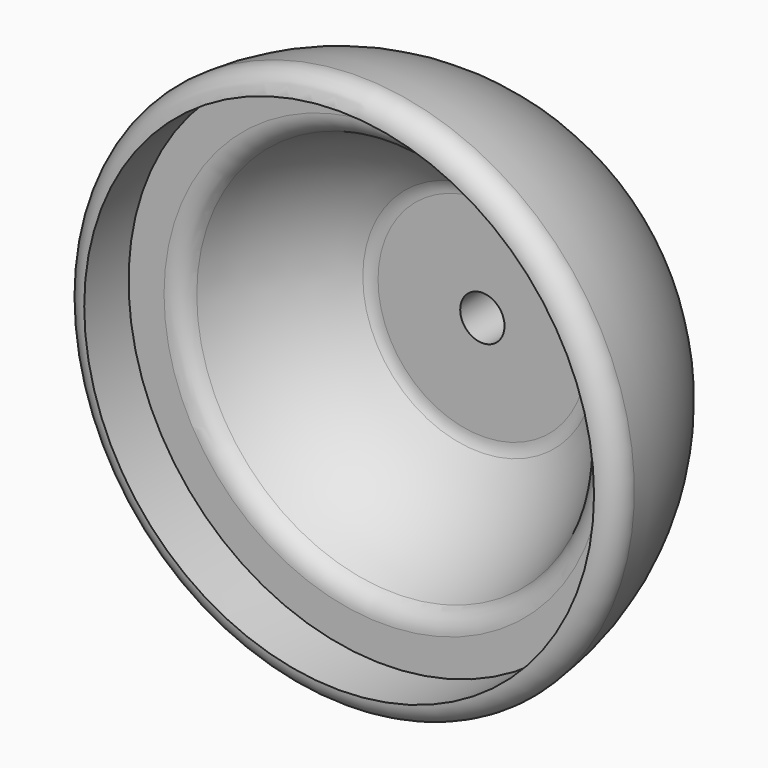
from build123d import *

# Parameters (mm, degrees)
F2_R      = 9
F2_R_2    = 6.5
F3_DEPTH  = 1
F4_R      = 5
F5_DEPTH  = 1
F6_R      = 23
F7_DEPTH  = 5
F8_R      = 2.5
F9_DEPTH  = 2
F10_R     = 2
F11_DEPTH = 25


# Not quite as in the source:
# - a fillet or chamfer that OpenCascade refuses, or shapes differently, is made with other operations: its cross-section is extruded or revolved along the edge and cut away or added


with BuildPart() as f1:
    # F0 (on Top) → F1 (revolve)
    with BuildSketch(Plane.XY):
        with BuildLine():
            ThreePointArc((-30.0702019767, 18.8458363465), (-40.98670264, 9.6260218093), (-45.0702019767, -4.0670421283))
            Line((-45.0702019767, -4.0670421283), (-39.0702019767, -4.0670421283))
            ThreePointArc((-39.0702019767, -4.0670421283), (-36.6683946494, 5.1795788761), (-30.0702019767, 12.0884522931))
            ThreePointArc((-30.0702019767, 12.0884522931), (-25.2685481557, 14.2080008813), (-20.0702019767, 14.9329578717))
            Line((-20.0702019767, 14.9329578717), (-20.0702019767, 18.8458363465))
            Line((-20.0702019767, 18.8458363465), (-30.0702019767, 18.8458363465))
        make_face()
        with BuildLine():
            ThreePointArc((-20.0702019767, 14.9329578717), (-25.2685481557, 14.2080008813), (-30.0702019767, 12.0884522931))
            Line((-30.0702019767, 12.0884522931), (-20.0702019767, 12.0884522931))
            Line((-20.0702019767, 12.0884522931), (-20.0702019767, 14.9329578717))
        make_face()
    revolve(axis=Axis((-20.0702019767, 9.4528388078, 0), (0, 1, 0)))

    # F2 (on face) → F3 (cut)
    with BuildSketch(Plane(origin=(0, 18.8458363465, 0), x_dir=(-1, 0, 0), z_dir=(0, 1, 0))):
        with Locations((20.0702019767, 0)):
            Circle(F2_R)
        with Locations((20.0702019767, 0)):
            Circle(F2_R_2, mode=Mode.SUBTRACT)
    extrude(amount=-F3_DEPTH, mode=Mode.SUBTRACT)

    # F4 (on face) → F5 (cut)
    with BuildSketch(Plane(origin=(0, 18.8458363465, 0), x_dir=(-1, 0, 0), z_dir=(0, 1, 0))):
        with Locations((20.0702019767, 0)):
            Circle(F4_R)
    extrude(amount=-F5_DEPTH, mode=Mode.SUBTRACT)

    # F6 (on face) → F7 (cut)
    with BuildSketch(Plane.XZ.offset(4.0670421283)):
        with Locations((-20.0702019767, 0)):
            Circle(F6_R)
    extrude(amount=-F7_DEPTH, mode=Mode.SUBTRACT)

    # F8 (on face) → F9 (join)
    with BuildSketch(Plane(origin=(0, 17.8458363465, 0), x_dir=(-1, 0, 0), z_dir=(0, 1, 0))):
        with Locations((20.0702019767, 0)):
            Circle(F8_R)
    extrude(amount=F9_DEPTH)

    # F10 (on face) → F11 (cut)
    with BuildSketch(Plane(origin=(0, 19.8458363465, 0), x_dir=(-1, 0, 0), z_dir=(0, 1, 0))):
        with Locations((20.0702019767, 0)):
            Circle(F10_R)
    extrude(amount=-F11_DEPTH, mode=Mode.SUBTRACT)

    # F12: fillet of radius 2 on 3 edges, made by hand

    # F12_s1 → F12_t2 (revolve)
    with BuildSketch(Plane.XY):
        with BuildLine():
            ThreePointArc((-30.5916471957, 11.753804578), (-30.0626140836, 12.0029632711), (-29.4841266463, 12.0884522931))
            Line((-29.4841266463, 12.0884522931), (-30.0702019767, 12.0884522931))
            ThreePointArc((-30.0702019767, 12.0884522931), (-30.3322887889, 11.9232541247), (-30.5916471957, 11.753804578))
        make_face()
    revolve(axis=Axis((-20.0702019767, 12.0884522931, 0), (0, 1, 0)))

    # F12_s3 → F12_t4 (revolve, cut)
    with BuildSketch(Plane.XY):
        with BuildLine():
            ThreePointArc((-44.9756840183, -1.895184795), (-44.4866456176, -3.3879435981), (-43.0702019767, -4.0670421283))
            Line((-43.0702019767, -4.0670421283), (-45.0702019767, -4.0670421283))
            ThreePointArc((-45.0702019767, -4.0670421283), (-45.0465613095, -2.9800856066), (-44.9756840183, -1.895184795))
        make_face()
    revolve(axis=Axis((-20.0702019767, -4.0670421283, 0), (0, 1, 0)), mode=Mode.SUBTRACT)

    # F12_s5 → F12_t6 (revolve, cut)
    with BuildSketch(Plane.XY):
        with BuildLine():
            ThreePointArc((-39.8691918499, 0.9329578717), (-38.7144913115, 1.2999647098), (-37.9835737667, 2.266291205))
            ThreePointArc((-37.9835737667, 2.266291205), (-38.2042977916, 1.6034577592), (-38.4005047565, 0.9329578717))
            Line((-38.4005047565, 0.9329578717), (-39.8691918499, 0.9329578717))
        make_face()
    revolve(axis=Axis((-20.0702019767, 0.9329578717, 0), (0, 1, 0)), mode=Mode.SUBTRACT)


solid = f1.part
